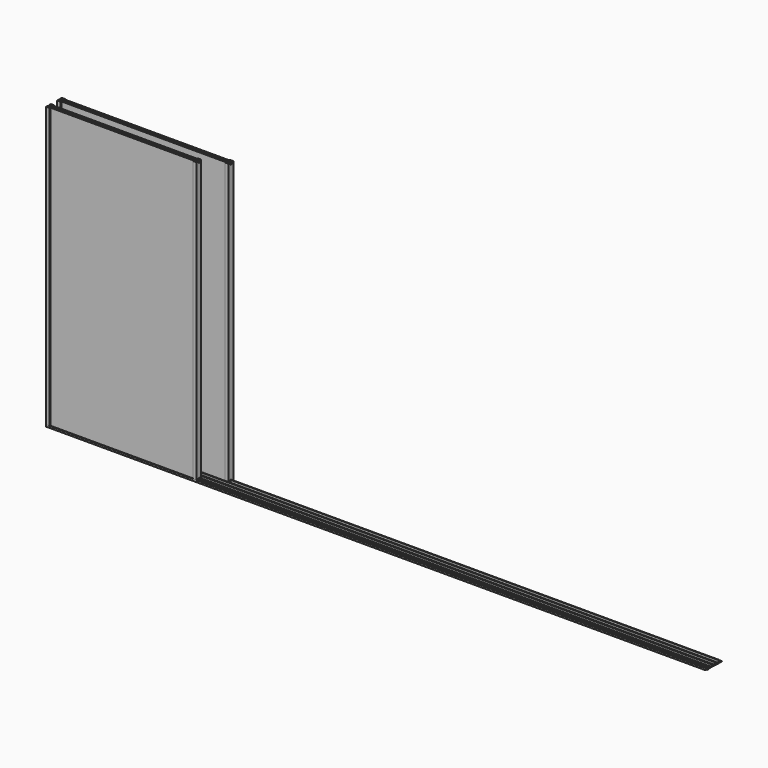
from build123d import *

# Parameters (mm, degrees)
F0_W     = 4.5
F0_H     = 9
F1_DEPTH = 4650
F2_DEPTH = 1210
F3_DEPTH = 25
F4_START = 1185
F4_DEPTH = 25
F5_DEPTH = 1060
F6_DEPTH = 25
F7_START = 1035
F7_DEPTH = 25


with BuildPart() as f1:
    # F0 (on Right) → F1 (new body)
    with BuildSketch(Plane.YZ):
        Polygon((-221, 4.2254131085), (-100, 0), (-100, 3.0018286329), (-125, 3.8748478702), (-125, 21), (-130, 21), (-130, 4.0494517176), (-157, 4.9923124939), (-157, 21), (-162, 21), (-162, 5.1669163414), (-189, 6.1097771177), (-189, 21), (-194, 21), (-194, 6.2843809651), (-221, 7.2272417414), (-221, 21), (-226, 21), (-226, 7.4018455889), (-240, 7.8907363617), (-240, 9), (-244.5, 9), (-244.5, 18), (-245, 18), (-245, 5.0635115763), (-226, 4.400016956), (-226, 0), (-221, 0), align=None)
        with Locations((-242.25, 13.5)):
            Rectangle(F0_W, F0_H)
    extrude(amount=F1_DEPTH)


with BuildPart() as f2:
    # F0 (on Right) → F2 (new body)
    with BuildSketch(Plane.YZ):
        Polygon((-132, 23), (-127.5, 23), (-123, 23), (-123, 9), (-112.5, 9), (-112.5, 1991), (-123, 1991), (-123, 1977), (-127.5, 1977), (-132, 1977), (-132, 1991), (-142.5, 1991), (-142.5, 9), (-132, 9), align=None)
    extrude(amount=F2_DEPTH)

    # F0 (on Right) → F3 (join)
    with BuildSketch(Plane.YZ):
        Polygon((-112.5, 1991), (-112.5, 9), (-106.5, 9), (-106.5, 1000), (-106.5, 1991), align=None)
        Polygon((-148.5, 9), (-142.5, 9), (-142.5, 1991), (-148.5, 1991), (-148.5, 1000), align=None)
    extrude(amount=F3_DEPTH)

    # F0 (on Right) → F4 (join)
    with BuildSketch(Plane.YZ.offset(F4_START)):
        Polygon((-112.5, 1991), (-112.5, 9), (-106.5, 9), (-106.5, 1000), (-106.5, 1991), align=None)
        Polygon((-148.5, 9), (-142.5, 9), (-142.5, 1991), (-148.5, 1991), (-148.5, 1000), align=None)
    extrude(amount=F4_DEPTH)


with BuildPart() as f5:
    # F0 (on Right) → F5 (new body)
    with BuildSketch(Plane.YZ):
        Polygon((-238.5, 1991), (-238.5, 9), (-228, 9), (-228, 23), (-223.5, 23), (-219, 23), (-219, 9), (-208.5, 9), (-208.5, 1991), (-219, 1991), (-219, 1977), (-223.5, 1977), (-228, 1977), (-228, 1991), align=None)
    extrude(amount=F5_DEPTH)

    # F0 (on Right) → F6 (join)
    with BuildSketch(Plane.YZ):
        Polygon((-208.5, 1991), (-208.5, 9), (-202.5, 9), (-202.5, 1000), (-202.5, 1991), align=None)
        Polygon((-244.5, 1000), (-244.5, 18), (-240, 18), (-240, 9), (-238.5, 9), (-238.5, 1991), (-244.5, 1991), align=None)
    extrude(amount=F6_DEPTH)

    # F0 (on Right) → F7 (join)
    with BuildSketch(Plane.YZ.offset(F7_START)):
        Polygon((-208.5, 1991), (-208.5, 9), (-202.5, 9), (-202.5, 1000), (-202.5, 1991), align=None)
        Polygon((-244.5, 1000), (-244.5, 18), (-240, 18), (-240, 9), (-238.5, 9), (-238.5, 1991), (-244.5, 1991), align=None)
    extrude(amount=F7_DEPTH)


solid = Compound([f1.part, f2.part, f5.part])
